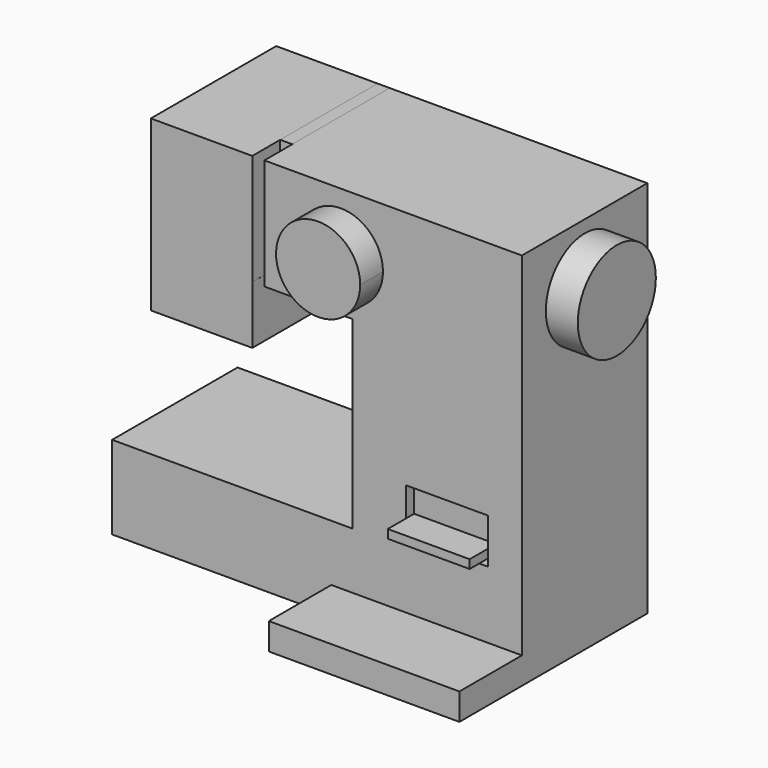
from build123d import *

# Parameters (mm, degrees)
F2_DEPTH = 76.2
F3_DEPTH = 90.03188
F0_W     = 39.8295894265
F0_H     = 14.2082143575
F0_H_2   = 3.4938193858
F4_DEPTH = 71.26206
F0_H_3   = 4.1925944388
F5_DEPTH = 87.27823
F0_W_2   = 92.7027892321
F0_H_4   = 13.0436122417
F6_DEPTH = 114.18662
F0_W_3   = 5.8787036687
F0_H_5   = 19.0941914916
F7_DEPTH = 59.22076
F1_R     = 23.7210403161
F8_DEPTH = 122.76001


with BuildPart() as f2:
    # F0 (on Front) → F2 (new body)
    with BuildSketch(Plane.XZ):
        Polygon((-73.2527300715, 87.5874310732), (-73.2527300715, 5.3862300701), (-23.8952767104, 5.3862300701), (-23.8952767104, 33.5842727341), (-23.9131078124, 33.5842727341), (-23.9131078124, 68.4932395816), (-23.9131078124, 87.5874310732), align=None)
    extrude(amount=F2_DEPTH)


with BuildPart() as f2b:
    # F0 (on Front) → F2, piece 2 (new body)
    with BuildSketch(Plane.XZ):
        Polygon((-18.0344041437, 68.4932395816), (-18.0344041437, 33.5842727341), (24.8745921999, 33.5842727341), (24.8745921999, -56.1147257686), (-92.0555666089, -56.1147257686), (-92.0555666089, -96.6535285115), (14.5113263279, -96.6535285115), (14.5113263279, -83.6099162698), (107.2141155601, -83.6099162698), (107.2141155601, 87.5874310732), (-18.0344041437, 87.5874310732), align=None)
        Polygon((90.6766802073, -51.0009080172), (50.8470907807, -51.0009080172), (50.8470907807, -47.5070886314), (50.8470907807, -43.3144941926), (50.8470907807, -29.1062798351), (90.6766802073, -29.1062798351), (90.6766802073, -43.3144941926), (90.6766802073, -47.5070886314), align=None, mode=Mode.SUBTRACT)
        with BuildLine():
            ThreePointArc((39.6350706735, 58.7051510811), (35.5340520557, 46.4153622337), (24.8745921999, 39.0510442613))
            ThreePointArc((24.8745921999, 39.0510442613), (2.8054622296, 70.9949399285), (39.6350706735, 58.7051510811))
        make_face(mode=Mode.SUBTRACT)
    extrude(amount=F2_DEPTH)

    # F0 (on Front) → F3 (join)
    with BuildSketch(Plane.XZ):
        with BuildLine():
            ThreePointArc((39.6350706735, 58.7051510811), (2.8054622296, 70.9949399285), (24.8745921999, 39.0510442613))
            ThreePointArc((24.8745921999, 39.0510442613), (35.5340520557, 46.4153622337), (39.6350706735, 58.7051510811))
        make_face()
    extrude(amount=F3_DEPTH)

    # F0 (on Front) → F4 (join)
    with BuildSketch(Plane.XZ):
        with Locations((70.761885494, -36.2103870139)):
            Rectangle(F0_W, F0_H)
        with Locations((70.761885494, -49.2539983243)):
            Rectangle(F0_W, F0_H_2)
    extrude(amount=F4_DEPTH)

    # F0 (on Front) → F5 (join)
    with BuildSketch(Plane.XZ):
        with Locations((70.761885494, -45.410791412)):
            Rectangle(F0_W, F0_H_3)
    extrude(amount=F5_DEPTH)

    # F0 (on Front) → F6 (join)
    with BuildSketch(Plane.XZ):
        with Locations((60.862720944, -90.1317223907)):
            Rectangle(F0_W_2, F0_H_4)
    extrude(amount=F6_DEPTH)

    # F1 (on Right) → F8 (join)
    with BuildSketch(Plane.YZ):
        with Locations((-37.9360765219, 57.8596889973)):
            Circle(F1_R)
    extrude(amount=F8_DEPTH)


with BuildPart() as f7:
    # F0 (on Front) → F7 (new body)
    with BuildSketch(Plane.XZ):
        with Locations((-20.973755978, 78.0403353274)):
            Rectangle(F0_W_3, F0_H_5)
    extrude(amount=F7_DEPTH)


solid = Compound([f2.part, f2b.part, f7.part])
